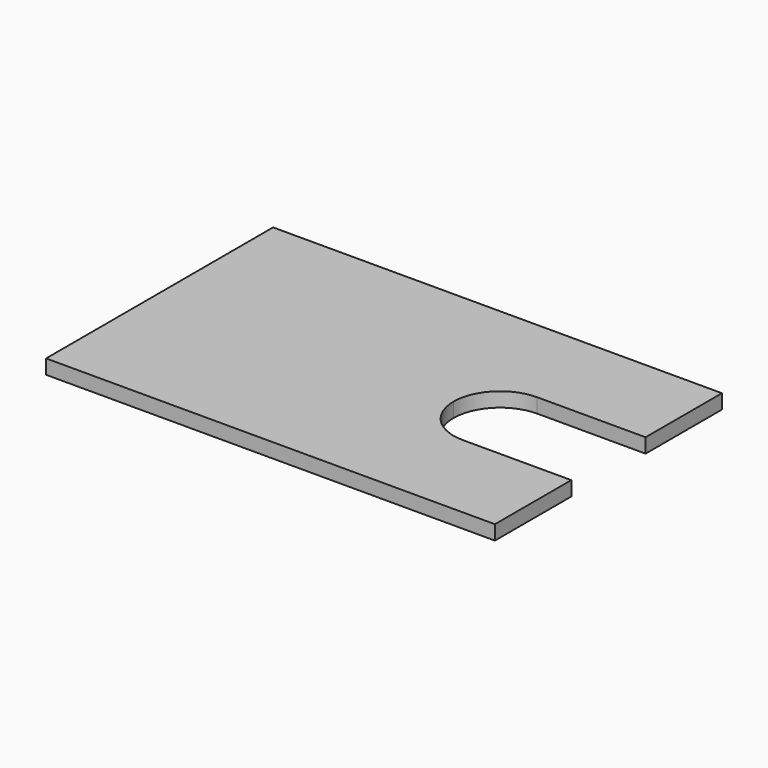
from build123d import *

# Parameters (mm, degrees)
F0_W     = 87
F0_H     = 55
F1_DEPTH = 2.8
F2_W     = 60
F2_H     = 18
F3_DEPTH = 25
F4_R     = 8.99999


# Not quite as in the source:
# - a fillet or chamfer is up to 0.001 mm smaller than in the source, because OpenCascade refuses the exact size


with BuildPart() as f1:
    # F0 (on Top) → F1 (new body)
    with BuildSketch(Plane.XY):
        Rectangle(F0_W, F0_H)
    extrude(amount=F1_DEPTH)

    # F2 (on face) → F3 (cut)
    with BuildSketch(Plane.XY.offset(2.8)):
        with Locations((43.5, 0)):
            Rectangle(F2_W, F2_H)
    extrude(amount=-F3_DEPTH, mode=Mode.SUBTRACT)

    # F4 (radius 9 in the source; OpenCascade refuses exactly that, so slightly less here)
    f4_edges = [f1.edges().sort_by_distance(p)[0] for p in [
        (13.5, 9, 1.4),
        (13.5, -9, 1.4),
    ]]
    fillet(f4_edges, radius=F4_R)


solid = f1.part
